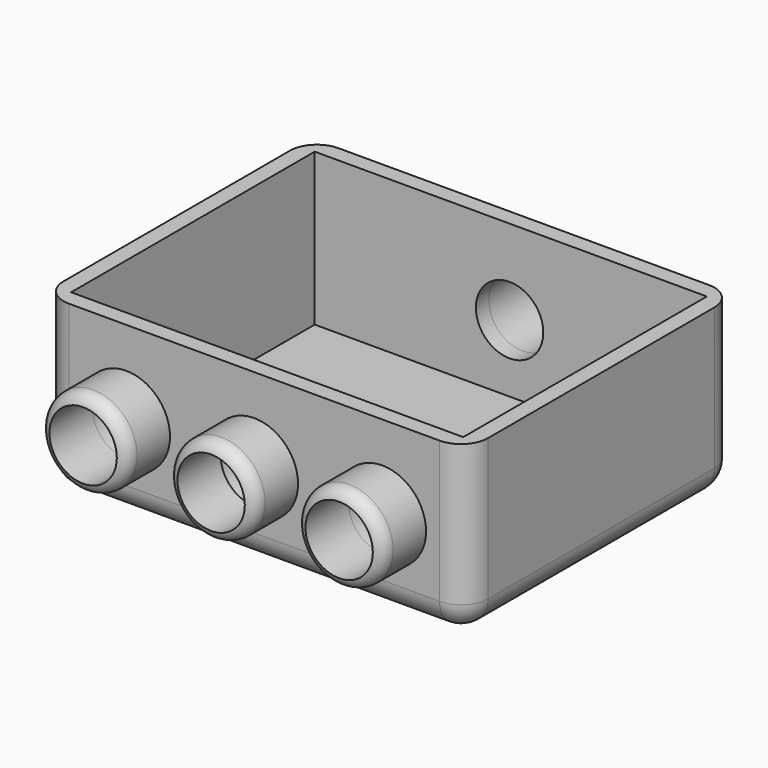
from build123d import *

# Parameters (mm, degrees)
F0_W     = 31.5
F0_H     = 12.5
F0_R     = 3.25
F0_R_2   = 2.5
F1_DEPTH = 25
F2_T     = -1.2
F3_R     = 3.25
F3_R_2   = 2.5
F4_DEPTH = 4
F5_DEPTH = 25
F6_DEPTH = 8
F7_DEPTH = 4
F8_R     = 2


# Not quite as in the source:
# - a fillet or chamfer that OpenCascade refuses, or shapes differently, is made with other operations: its cross-section is extruded or revolved along the edge and cut away or added


with BuildPart() as f1:
    # F0 (on Front) → F1 (new body)
    with BuildSketch(Plane.XZ):
        with Locations((-14.899123773, 20.1096497476)):
            Rectangle(F0_W, F0_H)
        with Locations((-24.399123773, 20.1096497476)):
            Circle(F0_R, mode=Mode.SUBTRACT)
        with Locations((-14.899123773, 20.1096497476)):
            Circle(F0_R, mode=Mode.SUBTRACT)
        with Locations((-5.399123773, 20.1096497476)):
            Circle(F0_R, mode=Mode.SUBTRACT)
        with Locations((-5.399123773, 20.1096497476)):
            Circle(F0_R)
        with Locations((-5.399123773, 20.1096497476)):
            Circle(F0_R_2, mode=Mode.SUBTRACT)
        with Locations((-14.899123773, 20.1096497476)):
            Circle(F0_R)
        with Locations((-14.899123773, 20.1096497476)):
            Circle(F0_R_2, mode=Mode.SUBTRACT)
        with Locations((-24.399123773, 20.1096497476)):
            Circle(F0_R)
        with Locations((-24.399123773, 20.1096497476)):
            Circle(F0_R_2, mode=Mode.SUBTRACT)
        with Locations((-5.399123773, 20.1096497476)):
            Circle(F0_R_2)
        with Locations((-14.899123773, 20.1096497476)):
            Circle(F0_R_2)
        with Locations((-24.399123773, 20.1096497476)):
            Circle(F0_R_2)
    extrude(amount=-F1_DEPTH)

    # F2
    f2_openings = [f1.faces().sort_by_distance(p)[0] for p in [
        (-14.899124, 12.5, 26.35965),
    ]]
    offset(amount=F2_T, openings=f2_openings)

    # F3 (on face) → F4 (join)
    with BuildSketch(Plane(origin=(0, 25, 0), x_dir=(-1, 0, 0), z_dir=(0, 1, 0))):
        with Locations((14.9896983057, 20.05478926)):
            Circle(F3_R)
        with Locations((14.9896983057, 20.05478926)):
            Circle(F3_R_2, mode=Mode.SUBTRACT)
    extrude(amount=F4_DEPTH)

    # F5 (cut): a face of the model
    f5_faces = [f1.faces().sort_by_distance(p)[0] for p in [
        (-14.9896983057, 25, 20.05478926),
    ]]
    extrude(f5_faces, amount=-F5_DEPTH, mode=Mode.SUBTRACT)

    # F0 (on Front) → F6 (cut)
    with BuildSketch(Plane.XZ):
        with Locations((-24.399123773, 20.1096497476)):
            Circle(F0_R_2)
        with Locations((-5.399123773, 20.1096497476)):
            Circle(F0_R_2)
    extrude(amount=-F6_DEPTH, mode=Mode.SUBTRACT)

    # F0 (on Front) → F7 (join)
    with BuildSketch(Plane.XZ):
        with Locations((-24.399123773, 20.1096497476)):
            Circle(F0_R)
        with Locations((-24.399123773, 20.1096497476)):
            Circle(F0_R_2, mode=Mode.SUBTRACT)
        with Locations((-14.899123773, 20.1096497476)):
            Circle(F0_R)
        with Locations((-14.899123773, 20.1096497476)):
            Circle(F0_R_2, mode=Mode.SUBTRACT)
        with Locations((-5.399123773, 20.1096497476)):
            Circle(F0_R)
        with Locations((-5.399123773, 20.1096497476)):
            Circle(F0_R_2, mode=Mode.SUBTRACT)
    extrude(amount=F7_DEPTH)

    # F8
    f8_edges = [f1.edges().sort_by_distance(p)[0] for p in [
        (0.850876, 12.5, 13.85965),
        (0.850876, 0, 20.10965),
        (-14.899124, 0, 13.85965),
        (-30.649124, 12.5, 13.85965),
        (-30.649124, 0, 20.10965),
        (-30.649124, 25, 20.10965),
        (-14.899124, 25, 13.85965),
        (0.850876, 25, 20.10965),
    ]]
    fillet(f8_edges, radius=F8_R)

    # F9: fillet of radius 1 on 4 edges, made by hand

    # F9_s1 → F9_t2 (revolve, cut)
    with BuildSketch(Plane.XY.offset(20.1096497476)):
        with BuildLine():
            ThreePointArc((-2.148723773, -3.0310064355), (-2.3582112834, -3.6439193102), (-2.8990234836, -4.0003872235))
            Line((-2.8990234836, -4.0003872235), (-2.8739168861, -4.0973253023))
            ThreePointArc((-2.8739168861, -4.0973253023), (-2.5240736283, -4.1001365685), (-2.149123773, -4.1001365685))
            Line((-2.149123773, -4.1001365685), (-2.0489872044, -4))
            ThreePointArc((-2.0489872044, -4), (-2.0489872044, -3.5155032177), (-2.0485872044, -3.0310064355))
            Line((-2.0485872044, -3.0310064355), (-2.148723773, -3.0310064355))
        make_face()
    revolve(axis=Axis((-5.399123773, -4, 20.1096497476), (0, -1, 0)), mode=Mode.SUBTRACT)

    # F9_s3 → F9_t4 (revolve, cut)
    with BuildSketch(Plane.XY.offset(20.1096497476)):
        with BuildLine():
            ThreePointArc((-11.648723773, -3.0310064355), (-11.8582112834, -3.6439193102), (-12.3990234836, -4.0003872235))
            Line((-12.3990234836, -4.0003872235), (-12.3739168861, -4.0973253023))
            ThreePointArc((-12.3739168861, -4.0973253023), (-12.0240736283, -4.1001365685), (-11.649123773, -4.1001365685))
            Line((-11.649123773, -4.1001365685), (-11.5489872044, -4))
            ThreePointArc((-11.5489872044, -4), (-11.5489872044, -3.5155032177), (-11.5485872044, -3.0310064355))
            Line((-11.5485872044, -3.0310064355), (-11.648723773, -3.0310064355))
        make_face()
    revolve(axis=Axis((-14.899123773, -4, 20.1096497476), (0, -1, 0)), mode=Mode.SUBTRACT)

    # F9_s5 → F9_t6 (revolve, cut)
    with BuildSketch(Plane.XY.offset(20.1096497476)):
        with BuildLine():
            ThreePointArc((-21.148723773, -3.0310064355), (-21.3582112834, -3.6439193102), (-21.8990234836, -4.0003872235))
            Line((-21.8990234836, -4.0003872235), (-21.8739168861, -4.0973253023))
            ThreePointArc((-21.8739168861, -4.0973253023), (-21.5240736283, -4.1001365685), (-21.149123773, -4.1001365685))
            Line((-21.149123773, -4.1001365685), (-21.0489872044, -4))
            ThreePointArc((-21.0489872044, -4), (-21.0489872044, -3.5155032177), (-21.0485872044, -3.0310064355))
            Line((-21.0485872044, -3.0310064355), (-21.148723773, -3.0310064355))
        make_face()
    revolve(axis=Axis((-24.399123773, -4, 20.1096497476), (0, -1, 0)), mode=Mode.SUBTRACT)

    # F9_s7 → F9_t8 (revolve, cut)
    with BuildSketch(Plane.XY.offset(20.05478926)):
        with BuildLine():
            ThreePointArc((-18.2400983057, 28.0310064355), (-18.0306107953, 28.6439193102), (-17.4897985952, 29.0003872235))
            Line((-17.4897985952, 29.0003872235), (-17.5149051926, 29.0973253023))
            ThreePointArc((-17.5149051926, 29.0973253023), (-17.8647484504, 29.1001365685), (-18.2396983057, 29.1001365685))
            Line((-18.2396983057, 29.1001365685), (-18.3398348743, 29))
            ThreePointArc((-18.3398348743, 29), (-18.3398348743, 28.5155032177), (-18.3402348743, 28.0310064355))
            Line((-18.3402348743, 28.0310064355), (-18.2400983057, 28.0310064355))
        make_face()
    revolve(axis=Axis((-14.9896983057, 29, 20.05478926), (0, 1, 0)), mode=Mode.SUBTRACT)


solid = f1.part
